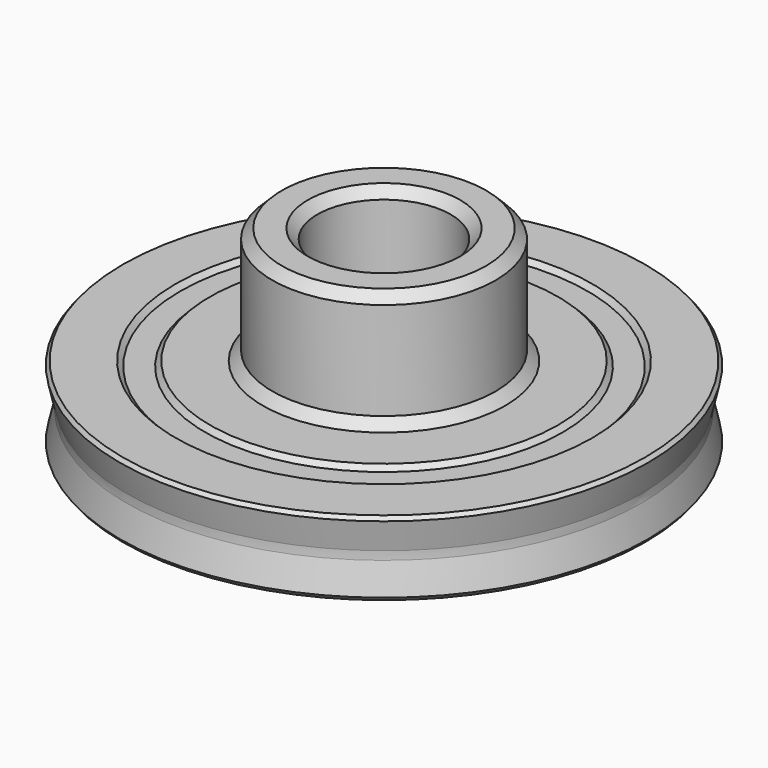
from build123d import *

# Parameters (mm, degrees)
F2_SIZE  = 0.2
F3_R     = 1
F4_SIZE  = 0.5
F5_SIZE  = 0.5
F6_R     = 11.6305905431
F6_R_2   = 8.3305905431
F7_DEPTH = 0.25


# Not quite as in the source:
# - a fillet or chamfer that OpenCascade refuses, or shapes differently, is made with other operations: its cross-section is extruded or revolved along the edge and cut away or added


with BuildPart() as f1:
    # F0 (on Front) → F1 (revolve)
    with BuildSketch(Plane.XZ):
        Polygon((5.8305905431, 10), (3.48, 10), (3.48, 0), (5.8305905431, 0), (13.8305905431, 0), (13.3861808223, 1.95), (13.8305905431, 3.9), (5.8305905431, 3.9), align=None)
    revolve(axis=Axis((0, 0, 13.5622331873), (0, 0, -1)))

    # F2
    f2_edges = [f1.edges().sort_by_distance(p)[0] for p in [
        (-13.830591, 0, 3.9),
        (-13.830591, 0, 0),
    ]]
    chamfer(f2_edges, length=F2_SIZE)

    # F3
    f3_edges = [f1.edges().sort_by_distance(p)[0] for p in [
        (-13.386181, 0, 1.95),
    ]]
    fillet(f3_edges, radius=F3_R)

    # F4
    f4_edges = [f1.edges().sort_by_distance(p)[0] for p in [
        (-5.830591, 0, 10),
        (-3.48, 0, 10),
        (-5.830591, 0, 3.9),
    ]]
    chamfer(f4_edges, length=F4_SIZE)

    # F5
    f5_edges = [f1.edges().sort_by_distance(p)[0] for p in [
        (-3.48, 0, 0),
    ]]
    chamfer(f5_edges, length=F5_SIZE)

    # F6 (on face) → F7 (cut)
    with BuildSketch(Plane.XY.offset(3.9)):
        Circle(F6_R)
        Circle(F6_R_2, mode=Mode.SUBTRACT)
    extrude(amount=-F7_DEPTH, mode=Mode.SUBTRACT)

    # F8: chamfer of 1 on 2 edges, made by hand


with BuildPart() as f8_tool2:
    # F8_s3 → F8_t4 (revolve)
    with BuildSketch(Plane.XZ):
        Polygon((10.6305905431, 3.65), (11.6305905431, 4.65), (11.6305905431, 3.65), align=None)
    revolve(axis=Axis((0, 0, 3.65), (0, 0, 1)))

    split(bisect_by=Plane.XY.offset(3.9), keep=Keep.BOTTOM)


with BuildPart() as f1_1:
    add(f1.part)

    # F8_t1: union F8_tool2
    add(f8_tool2.part)


with BuildPart() as f8_tool7:
    # F8_s8 → F8_t9 (revolve)
    with BuildSketch(Plane.XZ):
        Polygon((8.3305905431, 4.65), (9.3305905431, 3.65), (8.3305905431, 3.65), align=None)
    revolve(axis=Axis((0, 0, 3.65), (0, 0, 1)))

    split(bisect_by=Plane.XY.offset(3.9), keep=Keep.BOTTOM)


with BuildPart() as f1_2:
    add(f1_1.part)

    # F8_t6: union F8_tool7
    add(f8_tool7.part)


solid = f1_2.part
